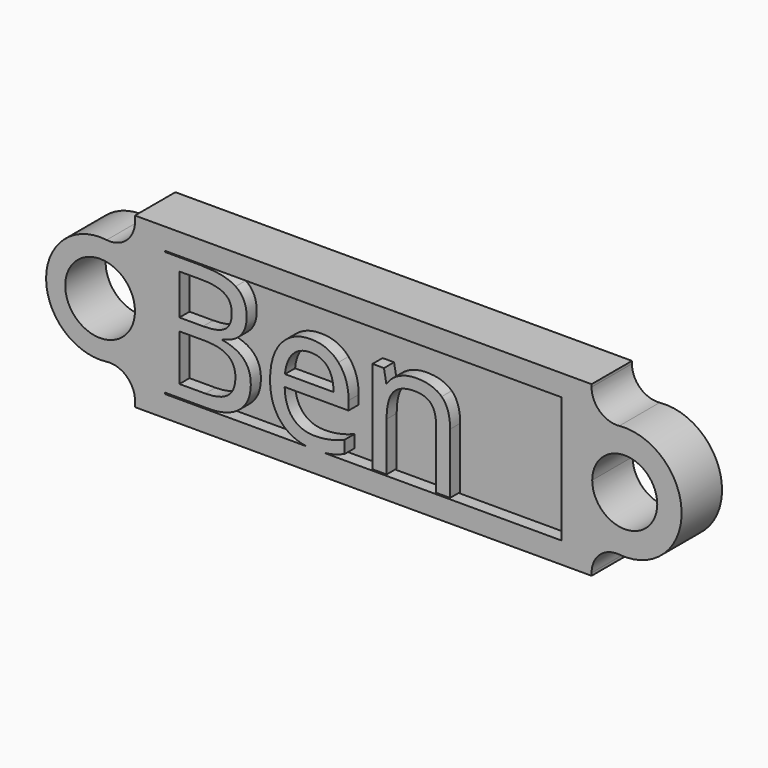
from build123d import *

# Parameters (mm, degrees)
F0_R     = 17.5342485309
F0_W     = 208.0285698175
F0_H     = 60.8816854656
F1_DEPTH = 25.4
F2_W     = 199.1405338049
F2_H     = 63.4146874705
F3_DEPTH = 6.35
F6_DEPTH = 6.35


with BuildPart() as f1:
    # F0 (on Front) → F1 (new body)
    with BuildSketch(Plane.XZ):
        with BuildLine():
            Line((114.7961392999, 41.1091820392), (114.7961392999, 42.4124971032))
            Line((114.7961392999, 42.4124971032), (-114.7961392999, 42.4124971032))
            Line((-114.7961392999, 42.4124971032), (-114.7961392999, 39.5639197406))
            ThreePointArc((-114.7961392999, 39.5639197406), (-119.0780712792, 30.0546542169), (-129.0364748589, 26.9576765903))
            ThreePointArc((-129.0364748589, 26.9576765903), (-159.4885576846, 0), (-129.0364748589, -26.9576765903))
            ThreePointArc((-129.0364748589, -26.9576765903), (-119.0780712792, -30.0546542169), (-114.7961392999, -39.5639197406))
            Line((-114.7961392999, -39.5639197406), (-114.7961392999, -42.4124971032))
            Line((-114.7961392999, -42.4124971032), (114.7961392999, -42.4124971032))
            Line((114.7961392999, -42.4124971032), (114.7961392999, -41.1091820392))
            ThreePointArc((114.7961392999, -41.1091820392), (118.9582568629, -31.7073437353), (128.7165429996, -28.4679552471))
            ThreePointArc((128.7165429996, -28.4679552471), (160.0651957896, 0), (128.7165429996, 28.4679552471))
            ThreePointArc((128.7165429996, 28.4679552471), (118.9582568629, 31.7073437353), (114.7961392999, 41.1091820392))
        make_face()
        with Locations((-132.3303878307, 0)):
            Circle(F0_R, mode=Mode.SUBTRACT)
        Rectangle(F0_W, F0_H, mode=Mode.SUBTRACT)
        with BuildLine():
            ThreePointArc((115.1127634511, 0), (131.4648836851, 16.352120234), (147.8170039192, 0))
            ThreePointArc((147.8170039192, 0), (131.4648836851, -16.352120234), (115.1127634511, 0))
        make_face(mode=Mode.SUBTRACT)
        Rectangle(F0_W, F0_H)
    extrude(amount=F1_DEPTH)

    # F2 (on face) → F3 (cut)
    with BuildSketch(Plane.XZ.offset(25.4)):
        Rectangle(F2_W, F2_H)
    extrude(amount=-F3_DEPTH, mode=Mode.SUBTRACT)

    # F4 (on face) → F6 (join)
    with BuildSketch(Plane.XZ.offset(19.05)):
        with BuildLine():
            Line((36.5855240286, -0.8747291355), (36.5855240286, -31.0594588518))
            Line((36.5855240286, -31.0594588518), (43.6549620804, -31.0594588518))
            Line((43.6549620804, -31.0594588518), (43.6549620804, -0.6295463129))
            add(Edge.make_bspline(
                [(39.3983158546, 12.3855751871), (43.6549620804, 8.3196267123), (43.6549620804, -0.6295463129)],
                knots=[0, 0, 0, 1, 1, 1], degree=2))
            add(Edge.make_bspline(
                [(26.7101047848, 16.451523662), (35.1416696288, 16.451523662), (39.3983158546, 12.3855751871)],
                knots=[0, 0, 0, 1, 1, 1], degree=2))
            add(Edge.make_bspline(
                [(17.9856826804, 14.5513567868), (21.9017972081, 16.451523662), (26.7101047848, 16.451523662)],
                knots=[0, 0, 0, 1, 1, 1], degree=2))
            add(Edge.make_bspline(
                [(11.890165285, 9.2050091272), (14.0695681526, 12.6511899116), (17.9856826804, 14.5513567868)],
                knots=[0, 0, 0, 1, 1, 1], degree=2))
            Line((11.890165285, 9.2050091272), (11.549633587, 9.2050091272))
            Line((11.549633587, 9.2050091272), (10.4054470815, 15.5933837829))
            Line((10.4054470815, 15.5933837829), (4.6572720182, 15.5933837829))
            Line((4.6572720182, 15.5933837829), (4.6572720182, -31.0594588518))
            Line((4.6572720182, -31.0594588518), (11.72671007, -31.0594588518))
            Line((11.72671007, -31.0594588518), (11.72671007, -6.582040395))
            add(Edge.make_bspline(
                [(15.1320270506, 6.4875661767), (11.72671007, 2.5305878452), (11.72671007, -6.582040395)],
                knots=[0, 0, 0, 1, 1, 1], degree=2))
            add(Edge.make_bspline(
                [(25.8519649056, 10.4445445082), (18.5373440312, 10.4445445082), (15.1320270506, 6.4875661767)],
                knots=[0, 0, 0, 1, 1, 1], degree=2))
            add(Edge.make_bspline(
                [(33.9906724894, 7.6317526822), (31.3958209501, 10.4445445082), (25.8519649056, 10.4445445082)],
                knots=[0, 0, 0, 1, 1, 1], degree=2))
            add(Edge.make_bspline(
                [(36.5855240286, -0.8747291355), (36.5855240286, 4.8189608562), (33.9906724894, 7.6317526822)],
                knots=[0, 0, 0, 1, 1, 1], degree=2))
        make_face()
        with BuildLine():
            Line((-82.0965833805, 31.1761142863), (-99.5702669024, 31.1761142863))
            Line((-99.5702669024, 31.1761142863), (-99.5702669024, -31.0594588518))
            Line((-99.5702669024, -31.0594588518), (-77.9693392, -31.0594588518))
            add(Edge.make_bspline(
                [(-62.1959109457, -26.3737426865), (-67.8351158656, -31.0594588518), (-77.9693392, -31.0594588518)],
                knots=[0, 0, 0, 1, 1, 1], degree=2))
            add(Edge.make_bspline(
                [(-56.5567060258, -13.3518105525), (-56.5567060258, -21.6880265211), (-62.1959109457, -26.3737426865)],
                knots=[0, 0, 0, 1, 1, 1], degree=2))
            add(Edge.make_bspline(
                [(-70.7364459331, 1.5498565548), (-56.5567060258, -0.8747291355), (-56.5567060258, -13.3518105525)],
                knots=[0, 0, 0, 1, 1, 1], degree=2))
            Line((-70.7364459331, 1.5498565548), (-70.7364459331, 1.9721158604))
            add(Edge.make_bspline(
                [(-61.7259772024, 6.6305894899), (-64.8111943868, 3.0345747583), (-70.7364459331, 1.9721158604)],
                knots=[0, 0, 0, 1, 1, 1], degree=2))
            add(Edge.make_bspline(
                [(-58.6407600179, 15.7704602659), (-58.6407600179, 10.2266042214), (-61.7259772024, 6.6305894899)],
                knots=[0, 0, 0, 1, 1, 1], degree=2))
            add(Edge.make_bspline(
                [(-64.1778054284, 27.4711294114), (-58.6407600179, 23.7661445364), (-58.6407600179, 15.7704602659)],
                knots=[0, 0, 0, 1, 1, 1], degree=2))
            add(Edge.make_bspline(
                [(-82.0965833805, 31.1761142863), (-69.7148508389, 31.1761142863), (-64.1778054284, 27.4711294114)],
                knots=[0, 0, 0, 1, 1, 1], degree=2))
        make_face()
        with BuildLine():
            Line((-92.4487470017, -24.8890244829), (-92.4487470017, -1.5966563354))
            Line((-92.4487470017, -1.5966563354), (-80.0533931921, -1.5966563354))
            add(Edge.make_bspline(
                [(-68.2028900995, -4.3209099199), (-72.0985727254, -1.5966563354), (-80.0533931921, -1.5966563354)],
                knots=[0, 0, 0, 1, 1, 1], degree=2))
            add(Edge.make_bspline(
                [(-64.3072074737, -12.8342023714), (-64.3072074737, -7.0451635044), (-68.2028900995, -4.3209099199)],
                knots=[0, 0, 0, 1, 1, 1], degree=2))
            add(Edge.make_bspline(
                [(-68.114351858, -21.9740731475), (-64.3072074737, -19.0591218121), (-64.3072074737, -12.8342023714)],
                knots=[0, 0, 0, 1, 1, 1], degree=2))
            add(Edge.make_bspline(
                [(-79.4540574036, -24.8890244829), (-71.9214962424, -24.8890244829), (-68.114351858, -21.9740731475)],
                knots=[0, 0, 0, 1, 1, 1], degree=2))
            Line((-79.4540574036, -24.8890244829), (-92.4487470017, -24.8890244829))
        make_face(mode=Mode.SUBTRACT)
        with BuildLine():
            Line((-80.5301375694, 4.5329142298), (-92.4487470017, 4.5329142298))
            Line((-92.4487470017, 4.5329142298), (-92.4487470017, 24.9103310419))
            Line((-92.4487470017, 24.9103310419), (-81.7969154862, 24.9103310419))
            add(Edge.make_bspline(
                [(-69.878306054, 22.5947154951), (-73.6241547327, 24.9103310419), (-81.7969154862, 24.9103310419)],
                knots=[0, 0, 0, 1, 1, 1], degree=2))
            add(Edge.make_bspline(
                [(-66.1324573753, 15.0349117981), (-66.1324573753, 20.2790999483), (-69.878306054, 22.5947154951)],
                knots=[0, 0, 0, 1, 1, 1], degree=2))
            add(Edge.make_bspline(
                [(-69.4969105522, 6.9370680181), (-66.1324573753, 9.3412218065), (-66.1324573753, 15.0349117981)],
                knots=[0, 0, 0, 1, 1, 1], degree=2))
            add(Edge.make_bspline(
                [(-80.5301375694, 4.5329142298), (-72.861363729, 4.5329142298), (-69.4969105522, 6.9370680181)],
                knots=[0, 0, 0, 1, 1, 1], degree=2))
        make_face(mode=Mode.SUBTRACT)
        with BuildLine():
            add(Edge.make_bspline(
                [(-28.1770388712, -31.7073437353), (-35.9783446463, -30.7660762397), (-40.8718160129, -25.6109516828)],
                knots=[0.1825887008, 0.1825887008, 0.1825887008, 1, 1, 1], degree=2))
            Line((-28.1770388712, -31.7073437353), (-19.8087642709, -31.7073437353))
            add(Edge.make_bspline(
                [(-16.4829357976, -31.209292799), (-18.0019268098, -31.5316908913), (-19.8087642709, -31.7073437353)],
                knots=[0, 0, 0, 0.4551678559, 0.4551678559, 0.4551678559], degree=2))
            add(Edge.make_bspline(
                [(-9.3998764779, -28.8936772521), (-13.1457251566, -30.500986867), (-16.4829357976, -31.209292799)],
                knots=[0, 0, 0, 1, 1, 1], degree=2))
            Line((-9.3998764779, -28.8936772521), (-9.3998764779, -22.587030204))
            add(Edge.make_bspline(
                [(-24.2879223172, -25.7335430941), (-16.7553611561, -25.7335430941), (-9.3998764779, -22.587030204)],
                knots=[0, 0, 0, 1, 1, 1], degree=2))
            add(Edge.make_bspline(
                [(-35.3756344062, -21.4768968683), (-31.4390879766, -25.7335430941), (-24.2879223172, -25.7335430941)],
                knots=[0, 0, 0, 1, 1, 1], degree=2))
            add(Edge.make_bspline(
                [(-39.5301211226, -9.0066260852), (-39.3121808358, -17.2202506425), (-35.3756344062, -21.4768968683)],
                knots=[0, 0, 0, 1, 1, 1], degree=2))
            Line((-39.5301211226, -9.0066260852), (-7.3975500933, -9.0066260852))
            Line((-7.3975500933, -9.0066260852), (-7.3975500933, -4.5388502066))
            add(Edge.make_bspline(
                [(-12.5055255642, 10.6829166968), (-7.3975500933, 4.9143097316), (-7.3975500933, -4.5388502066)],
                knots=[0, 0, 0, 1, 1, 1], degree=2))
            add(Edge.make_bspline(
                [(-26.3719763094, 16.451523662), (-17.6135010352, 16.451523662), (-12.5055255642, 10.6829166968)],
                knots=[0, 0, 0, 1, 1, 1], degree=2))
            add(Edge.make_bspline(
                [(-41.3008859525, 9.8111555498), (-35.7434086401, 16.451523662), (-26.3719763094, 16.451523662)],
                knots=[0, 0, 0, 1, 1, 1], degree=2))
            add(Edge.make_bspline(
                [(-46.8583632649, -8.1212436702), (-46.8583632649, 3.1707874375), (-41.3008859525, 9.8111555498)],
                knots=[0, 0, 0, 1, 1, 1], degree=2))
            add(Edge.make_bspline(
                [(-40.8718160129, -25.6109516828), (-46.8583632649, -19.3043046347), (-46.8583632649, -8.1212436702)],
                knots=[0, 0, 0, 1, 1, 1], degree=2))
        make_face()
        with BuildLine():
            add(Edge.make_bspline(
                [(-26.4673251849, 10.5262721157), (-32.0792875689, 10.5262721157), (-35.4233088439, 6.8689616785)],
                knots=[0, 0, 0, 1, 1, 1], degree=2))
            add(Edge.make_bspline(
                [(-17.9472220993, 6.9711211879), (-20.9234691404, 10.5262721157), (-26.4673251849, 10.5262721157)],
                knots=[0, 0, 0, 1, 1, 1], degree=2))
            add(Edge.make_bspline(
                [(-14.9709750582, -3.2584510219), (-14.9709750582, 3.4159702601), (-17.9472220993, 6.9711211879)],
                knots=[0, 0, 0, 1, 1, 1], degree=2))
            Line((-14.9709750582, -3.2584510219), (-39.3666659075, -3.2584510219))
            add(Edge.make_bspline(
                [(-35.4233088439, 6.8689616785), (-38.7673301189, 3.2116512413), (-39.3666659075, -3.2584510219)],
                knots=[0, 0, 0, 1, 1, 1], degree=2))
        make_face(mode=Mode.SUBTRACT)
    extrude(amount=F6_DEPTH)


solid = f1.part
